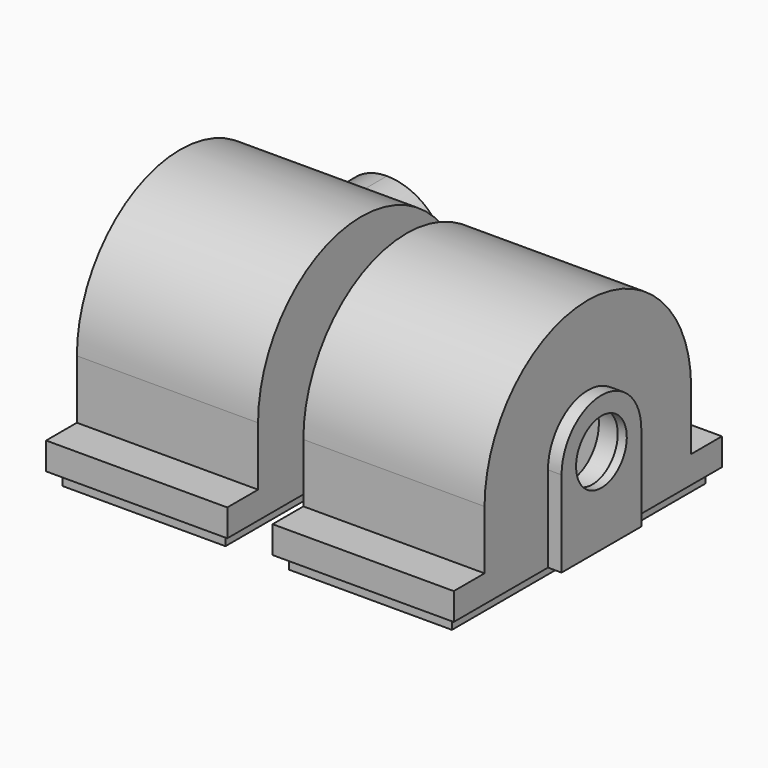
from build123d import *

# Parameters (mm, degrees)
F1_DEPTH  = 20
F3_DEPTH  = 16
F5_DEPTH  = 3
F8_W      = 36
F8_H      = 70
F9_DEPTH  = 3
F13_DEPTH = 11
F14_R     = 10.99999
F18_DEPTH = 11
F21_R     = 10.99999


# Not quite as in the source:
# - a fillet or chamfer is up to 0.001 mm smaller than in the source, because OpenCascade refuses the exact size
# - a pattern or mirror of a feature is missing from the dataset's text; its kind, count and spacing are read off the source's solid


with BuildPart() as f1:
    # F0 (on Right) → F1 (new body, symmetric)
    with BuildSketch(Plane.YZ):
        with BuildLine():
            Line((28.5, 9), (28.5, 22))
            ThreePointArc((28.5, 22), (0, 50.5), (-28.5, 22))
            Line((-28.5, 22), (-28.5, 9))
            Line((-28.5, 9), (-37, 9))
            Line((-37, 9), (-37, 0))
            Line((-37, 0), (37, 0))
            Line((37, 0), (37, 9))
            Line((37, 9), (28.5, 9))
        make_face()
    extrude(amount=F1_DEPTH, both=True)

    # F2 (on Right) → F3 (cut, symmetric)
    with BuildSketch(Plane.YZ):
        with BuildLine():
            Line((24.5, 0), (24.5, 22))
            ThreePointArc((24.5, 22), (0, 46.5), (-24.5, 22))
            Line((-24.5, 22), (-24.5, 0))
            Line((-24.5, 0), (24.5, 0))
        make_face()
    extrude(amount=F3_DEPTH, both=True, mode=Mode.SUBTRACT)

    # F4 (on face) → F5 (join)
    with BuildSketch(Plane.YZ.offset(20)):
        with BuildLine():
            Line((11, 0), (11, 22))
            ThreePointArc((11, 22), (0, 33), (-11, 22))
            Line((-11, 22), (-11, 0))
            Line((-11, 0), (11, 0))
        make_face()
    f5 = extrude(amount=F5_DEPTH)

    # F5_copies: F5 across plane
    add(f5.mirror(Plane(origin=(0, 0, 0), x_dir=(0, 0, -1), z_dir=(-1, 0, 0))))

    # F6 (on Front) → F7 (revolve, cut)
    with BuildSketch(Plane.XZ):
        Polygon((16, 30.05), (16, 22), (23, 22), (23, 29), (21, 29), (21, 30.05), align=None)
    f7 = revolve(axis=Axis((24.6842799243, 0, 22), (-1, 0, 0)), mode=Mode.SUBTRACT)

    # F7_copies: F7 across plane
    add(f7.mirror(Plane(origin=(0, 0, 0), x_dir=(0, 0, -1), z_dir=(-1, 0, 0))), mode=Mode.SUBTRACT)

    # F8 (on face) → F9 (cut)
    with BuildSketch(Plane(origin=(0, 0, 0), x_dir=(1, 0, 0), z_dir=(0, 0, -1))):
        Polygon((20, 37), (-20, 37), (-20, 11), (-23, 11), (-23, -11), (-20, -11), (-20, -37), (20, -37), (20, -11), (23, -11), (23, 11), (20, 11), align=None)
        Rectangle(F8_W, F8_H, mode=Mode.SUBTRACT)
    extrude(amount=-F9_DEPTH, mode=Mode.SUBTRACT)


with BuildPart() as f10_1:
    # F10: copy of F1
    add(f1.part.moved(Location((50, 0, 0))))

    # F12 (on mid) → F13 (join, symmetric)
    with BuildSketch(Plane.YZ.offset(50)):
        Polygon((21.5, 33), (21.5, 0), (34.5, 0), (34.5, 33), (24.8438753188, 33), (21.5, 34), align=None)
    extrude(amount=F13_DEPTH, both=True)

    # F14 (radius 11 in the source; OpenCascade refuses exactly that, so slightly less here)
    f14_edges = [f10_1.edges().sort_by_distance(p)[0] for p in [
        (61, 30.395817, 33),
        (39, 30.395817, 33),
    ]]
    fillet(f14_edges, radius=F14_R)

    # F15 (on mid) → F16 (revolve, cut)
    with BuildSketch(Plane.YZ.offset(50)):
        Polygon((21.5, 30), (21.5, 22), (34.5, 22), (34.5, 30), (29.5, 30), (29.5, 27.5), (26.5, 27.5), (26.5, 30), align=None)
    revolve(axis=Axis((50, 24.9189473689, 22), (0, 1, 0)), mode=Mode.SUBTRACT)


with BuildPart() as f1_1:
    add(f1.part)

    # F17 (on Right) → F18 (join, symmetric)
    with BuildSketch(Plane.YZ):
        with BuildLine():
            Line((21.5, 22), (21.5, 0))
            Line((21.5, 0), (34.5, 0))
            Line((34.5, 0), (34.5, 22))
            ThreePointArc((34.5, 22), (34.3687170842, 25.0068731248), (33.9758674789, 27.9908621295))
            Line((33.9758674789, 27.9908621295), (32.0657375246, 38.8237474126))
            Line((32.0657375246, 38.8237474126), (18.8651915701, 38.8237474126))
            Line((18.8651915701, 38.8237474126), (21.1733666898, 25.7334358198))
            ThreePointArc((21.1733666898, 25.7334358198), (21.418186009, 23.8738484691), (21.5, 22))
        make_face()
    extrude(amount=F18_DEPTH, both=True)

    # F19 (on Right) → F20 (revolve, cut)
    with BuildSketch(Plane.YZ):
        Polygon((27.6626432925, 35.0010832653), (28.1835878255, 32.0466600062), (25.2291645665, 31.5257154732), (24.7082200335, 34.4801387323), (19.7841812684, 33.6118978439), (16.8297580094, 33.0909533109), (18.2189434307, 25.2124912868), (21.1733666898, 25.7334358198), (33.9758674789, 27.9908621295), (32.5866820576, 35.8693241536), align=None)
    revolve(axis=Axis((0, 21.387808256, 25.7712476538), (0, 0.984807753, 0.1736481777)), mode=Mode.SUBTRACT)

    # F21 (radius 11 in the source; OpenCascade refuses exactly that, so slightly less here)
    f21_edges = [f1_1.edges().sort_by_distance(p)[0] for p in [
        (-11, 27.535168, 38.823747),
        (11, 27.535168, 38.823747),
    ]]
    fillet(f21_edges, radius=F21_R)


solid = Compound([f10_1.part, f1_1.part])
